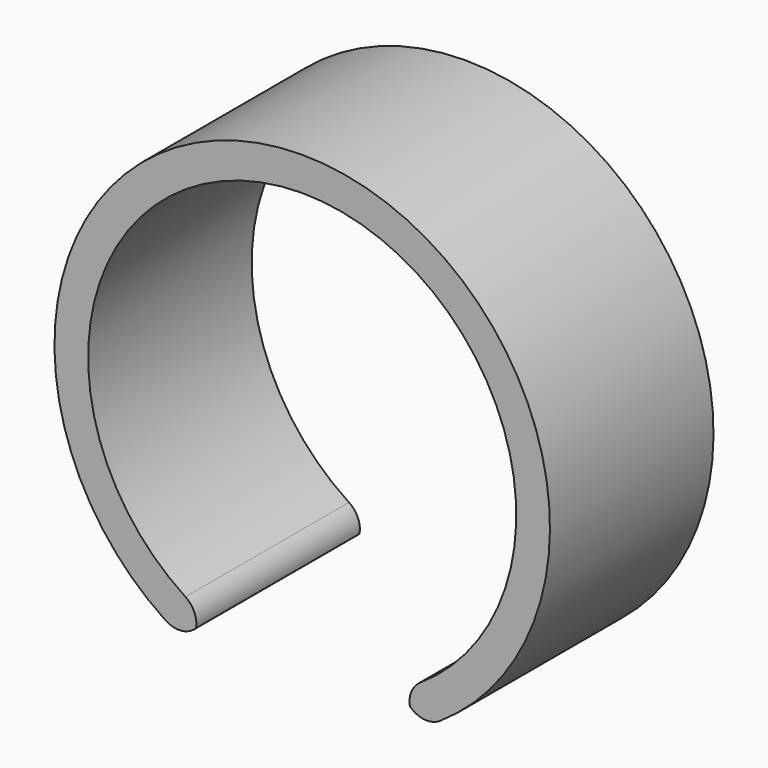
from build123d import *

# Parameters (mm, degrees)
F1_DEPTH    = 8.5
F2_T1_DEPTH = 13.246827309
F2_T3_DEPTH = 14.0456784574


# Not quite as in the source:
# - a fillet or chamfer that OpenCascade refuses, or shapes differently, is made with other operations: its cross-section is extruded or revolved along the edge and cut away or added


with BuildPart() as f1:
    # F0 (on Front) → F1 (new body)
    with BuildSketch(Plane.XZ):
        with BuildLine():
            ThreePointArc((-4.0781486701, -7.910670226), (-0.0323602773, 8.899941169), (4.1355666361, -7.880805073))
            Line((4.1355666361, -7.880805073), (4.7861052081, -9.1204822755))
            ThreePointArc((4.7861052081, -9.1204822755), (-0.037450658, 10.2999319147), (-4.7196552025, -9.1550453177))
            Line((-4.7196552025, -9.1550453177), (-4.0781486701, -7.910670226))
        make_face()
    extrude(amount=F1_DEPTH)

    # F2: fillet of radius 1 on 4 edges, made by hand

    # F2_s2 → F2_t1 (cut)
    with BuildSketch(Plane.XZ.offset(-2.3734136545)):
        with BuildLine():
            ThreePointArc((-4.8563481702, -7.4582761044), (-4.4353117021, -8.0403480428), (-4.5131659168, -8.7545036072))
            Line((-4.5131659168, -8.7545036072), (-4.0781486701, -7.910670226))
            ThreePointArc((-4.0781486701, -7.910670226), (-4.4729714461, -7.6943178023), (-4.8563481702, -7.4582761044))
        make_face()
        with BuildLine():
            ThreePointArc((4.9104557842, -7.4227639051), (4.4936632318, -8.0078821984), (4.5767086731, -8.72145273))
            Line((4.5767086731, -8.72145273), (4.1355666361, -7.880805073))
            ThreePointArc((4.1355666361, -7.880805073), (4.5288056742, -7.6615872484), (4.9104557842, -7.4227639051))
        make_face()
    extrude(amount=F2_T1_DEPTH, mode=Mode.SUBTRACT)

    # F2_s4 → F2_t3 (cut)
    with BuildSketch(Plane.XZ.offset(-2.7728392287)):
        with BuildLine():
            ThreePointArc((4.2963798875, -8.1872534993), (4.9361379588, -8.6919225089), (5.7390532384, -8.5529683693))
            ThreePointArc((5.7390532384, -8.5529683693), (5.2702237229, -8.849561679), (4.7861052081, -9.1204822755))
            Line((4.7861052081, -9.1204822755), (4.2963798875, -8.1872534993))
        make_face()
        with BuildLine():
            ThreePointArc((-5.6767049543, -8.5944761831), (-4.8728004404, -8.7275879094), (-4.2367291997, -8.2182799714))
            Line((-4.2367291997, -8.2182799714), (-4.7196552025, -9.1550453177))
            ThreePointArc((-4.7196552025, -9.1550453177), (-5.2057310309, -8.8876523579), (-5.6767049543, -8.5944761831))
        make_face()
    extrude(amount=F2_T3_DEPTH, mode=Mode.SUBTRACT)


solid = f1.part
